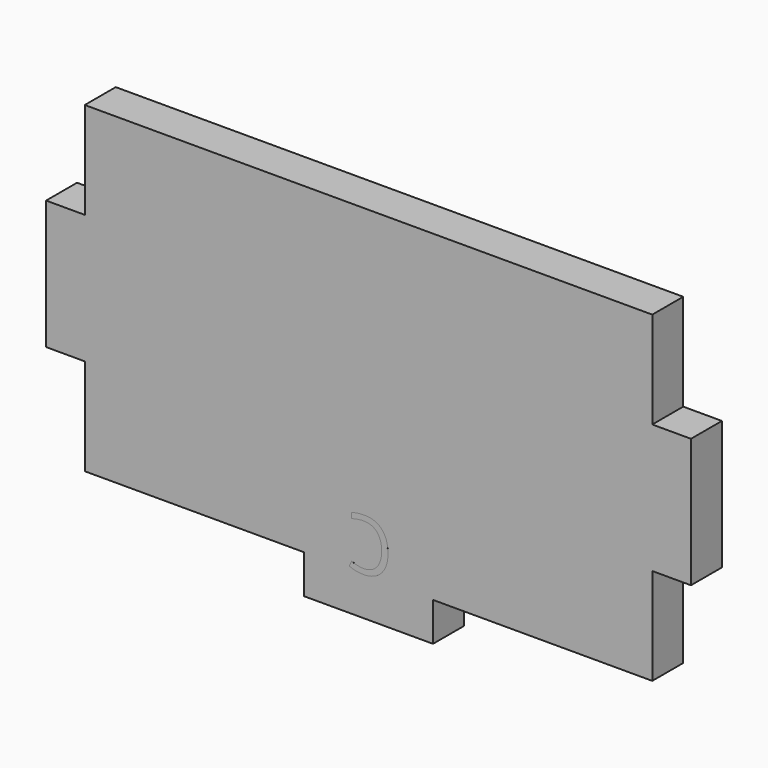
from build123d import *

# Parameters (mm, degrees)
F0_W         = 10
F0_H         = 3
F0_W_2       = 3
F0_H_2       = 10
F1_DEPTH     = 3
F2_TEXT_SIZE = 5.5555555556
F3_DEPTH     = 0.001


# Not quite as in the source:
# - Text() gives the source's letters only with a copy of the font that has no kerning and outlines rounded to 1/6400 em; it was checked with that copy


with BuildPart() as f1:
    # F0 (on Front) → F1 (new body)
    with BuildSketch(Plane.XZ):
        Polygon((-17, 0), (0, 0), (0, 7.5), (0, 17.5), (0, 25), (-44, 25), (-44, 17.5), (-44, 7.5), (-44, 0), (-27, 0), align=None)
        with Locations((-22, -1.5)):
            Rectangle(F0_W, F0_H)
        with Locations((1.5, 12.5)):
            Rectangle(F0_W_2, F0_H_2)
        with Locations((-45.5, 12.5)):
            Rectangle(F0_W_2, F0_H_2)
    extrude(amount=F1_DEPTH)

    # F2 (on face) → F3 (join)
    with BuildSketch(Plane.XZ.offset(3)):
        with Locations(Location((-20.1501736111, 4), (0, 0, 180))):
            Text('C', F2_TEXT_SIZE, font='Open Sans', text_align=(TextAlign.LEFT, TextAlign.BOTTOM))
    extrude(amount=F3_DEPTH)


solid = f1.part
